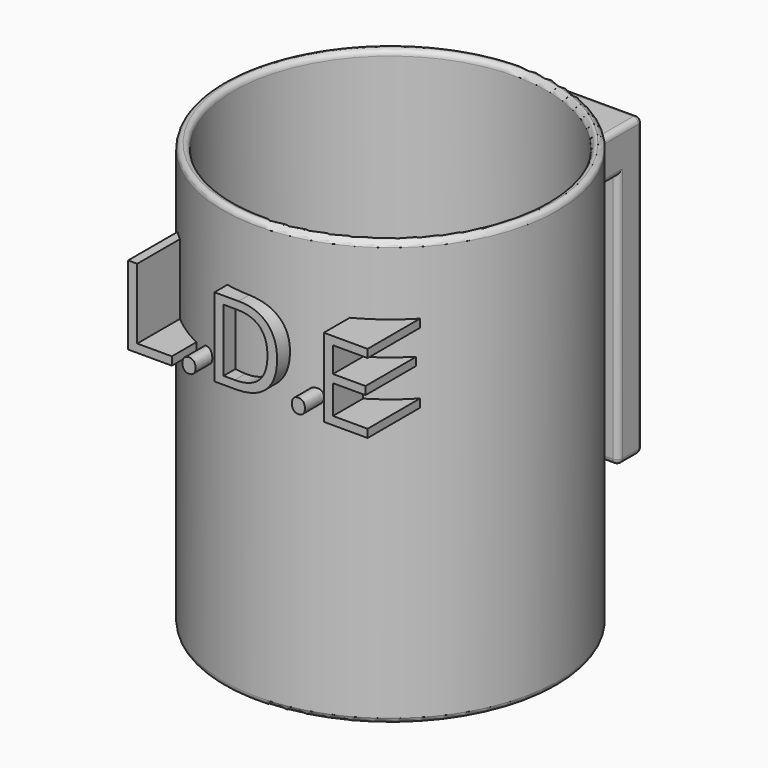
from build123d import *

# Parameters (mm, degrees)
F1_R          = 40.0234749814
F2_DEPTH      = 101.6
F3_T          = -2.54
F4_R          = 1.26999
F6_W          = 9.4942720607
F6_H          = 9.9551621825
F7_DEPTH      = 25.4
F8_W          = 18.9885441214
F8_H          = 7.3389949501
F9_DEPTH      = 60.96
F10_R         = 1.27
F12_TEXT_SIZE = 26.2893188906


# Not quite as in the source:
# - a fillet or chamfer is up to 0.001 mm smaller than in the source, because OpenCascade refuses the exact size
# - Text() gives the source's letters only with a copy of the font that has no kerning and outlines rounded to 1/6400 em; it was checked with that copy


with BuildPart() as f2:
    # F1 (on offset) → F2 (new body)
    with BuildSketch(Plane.XY.offset(43.18)):
        Circle(F1_R)
    extrude(amount=-F2_DEPTH)

    # F3
    f3_openings = [f2.faces().sort_by_distance(p)[0] for p in [
        (0, 0, 43.18),
    ]]
    offset(amount=F3_T, openings=f3_openings)

    # F4 (radius 1.27 in the source; OpenCascade refuses exactly that, so slightly less here)
    f4_edges = [f2.edges().sort_by_distance(p)[0] for p in [
        (-37.483475, 0, 43.18),
        (-40.023475, 0, 43.18),
        (-40.023475, 0, -58.42),
    ]]
    fillet(f4_edges, radius=F4_R)

    # F6 (on offset) → F7 (join)
    with BuildSketch(Plane.XZ.offset(-63.5)):
        with Locations((4.7471360303, 21.1086301133)):
            Rectangle(F6_W, F6_H)
        with Locations((-4.7471360303, 21.1086301133)):
            Rectangle(F6_W, F6_H)
    extrude(amount=F7_DEPTH)

    # F8 (on face) → F9 (join)
    with BuildSketch(Plane(origin=(0, 0, 16.1310490221), x_dir=(1, 0, 0), z_dir=(0, 0, -1))):
        with Locations((0, -59.830502525)):
            Rectangle(F8_W, F8_H)
    extrude(amount=F9_DEPTH)

    # F10
    f10_edges = [f2.edges().sort_by_distance(p)[0] for p in [
        (0, 63.5, 26.086211),
        (9.494272, 51.190533, 26.086211),
        (9.494272, 63.5, -9.37137),
        (9.494272, 59.830503, -44.828951),
        (9.494272, 56.161005, -14.348951),
        (9.494272, 47.521036, 16.131049),
        (9.494272, 38.881067, 21.10863),
        (-9.494272, 63.5, -9.37137),
        (-9.494272, 47.521036, 16.131049),
        (-9.494272, 51.190533, 26.086211),
        (0, 63.5, -44.828951),
        (0, 56.161005, -44.828951),
        (-9.494272, 59.830503, -44.828951),
        (0, 40.023475, 16.131049),
        (-9.494272, 38.881067, 21.10863),
        (0, 40.023475, 26.086211),
        (-9.494272, 56.161005, -14.348951),
    ]]
    fillet(f10_edges, radius=F10_R)


with BuildPart() as f13:
    # F12 (on offset) → F13 (new body, up to the next surface of F2)
    with BuildSketch(Plane.XZ.offset(43.18)):
        with Locations((-30.7749339263, 8.0194347538)):
            Text('L.D.E', F12_TEXT_SIZE, font='Open Sans', text_align=(TextAlign.LEFT, TextAlign.BOTTOM))
    extrude(until=Until.NEXT, target=f2.part, dir=(0, 1, 0))


solid = Compound([f2.part, f13.part])
